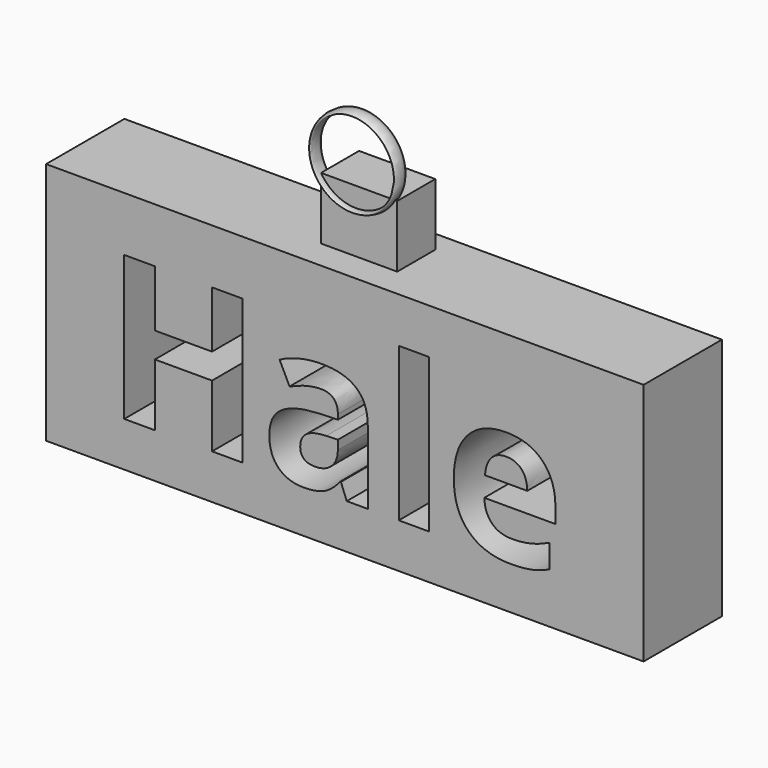
from build123d import *

# Parameters (mm, degrees)
F0_W         = 29.7667570412
F0_H         = 12.1342204511
F1_DEPTH     = 4.8768
F3_W         = 3.7970170379
F3_H         = 2.3699097801
F4_DEPTH     = 3.0988
F6_R         = 0.345188964
F2_TEXT_SIZE = 10.0751873106
F8_DEPTH     = 25.4


# Not quite as in the source:
# - Text() gives the source's letters only with a copy of the font that has no kerning and outlines rounded to 1/6400 em; it was checked with that copy


with BuildPart() as f1:
    # F0 (on Front) → F1 (new body)
    with BuildSketch(Plane.XZ):
        with Locations((-54.7935795039, 60.3866968304)):
            Rectangle(F0_W, F0_H)
    extrude(amount=-F1_DEPTH)

    # F3 (on face) → F4 (join)
    with BuildSketch(Plane.XY.offset(66.453807056)):
        with Locations((-55.2476122975, 2.6407511905)):
            Rectangle(F3_W, F3_H)
    extrude(amount=F4_DEPTH)

    # F7: sweep along a path in F5
    with BuildLine(Plane.XZ.offset(-1.4557963004)) as f7_path:
        CenterArc((-55.3914681077, 70.6199780107), 2.3853215303, 0, 360)
    # F6 (on face) → F7 (sweep)
    with BuildSketch(Plane.YZ.offset(-53.3491037786)):
        with Locations((1.5243095113, 71.1432471871)):
            Circle(F6_R)
    sweep(path=f7_path.line)

    # F2 (on face) → F8 (cut)
    with BuildSketch(Plane.XZ):
        with Locations((-66.688388586, 56.5432347357)):
            Text('Hale', F2_TEXT_SIZE, font='Open Sans', font_style=FontStyle.BOLD, text_align=(TextAlign.LEFT, TextAlign.BOTTOM))
    extrude(amount=-F8_DEPTH, mode=Mode.SUBTRACT)


solid = f1.part
